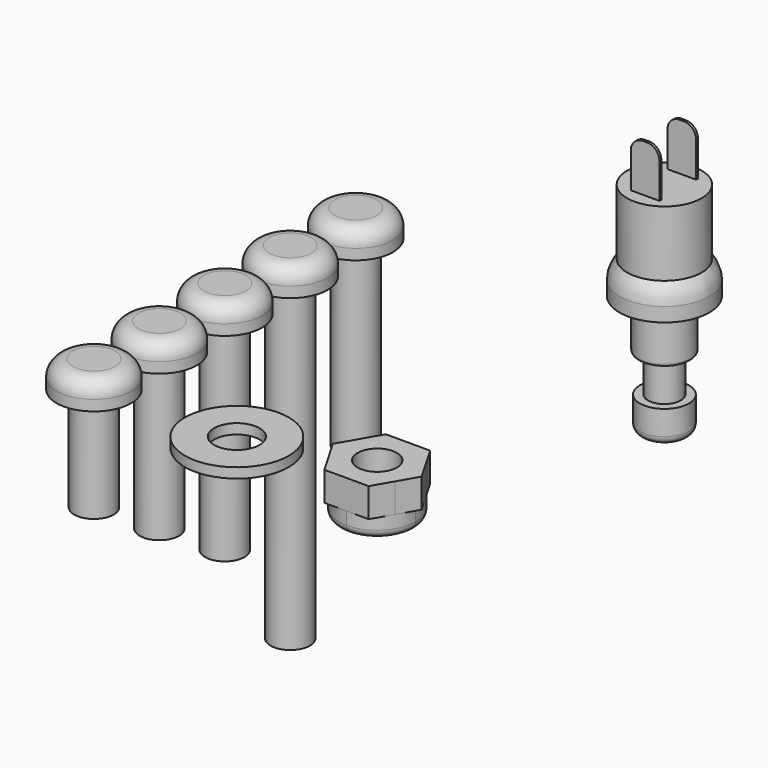
from build123d import *

# Parameters (mm, degrees)
F0_R      = 3
F1_DEPTH  = 4
F2_R      = 2
F3_DEPTH  = 4.6
F4_R      = 3.175
F5_DEPTH  = 6
F6_R      = 5.5
F7_DEPTH  = 4
F8_R      = 4.5612364212
F9_DEPTH  = 8
F11_R     = 1
F12_R     = 0.3
F13_W     = 3.5
F13_H     = 0.3
F14_DEPTH = 5.8
F15_R     = 1.5
F16_R     = 4.57
F16_R_2   = 2.413
F17_DEPTH = 3.3
F18_R     = 2
F19_DEPTH = 1
F21_DEPTH = 11.7
F23_DEPTH = 18.05
F25_DEPTH = 24.4
F27_DEPTH = 38
F28_R     = 6.35
F28_R_2   = 2.78
F29_DEPTH = 1.225
F30_R     = 2.413
F31_DEPTH = 3.56
F32_DEPTH = 2.54
F33_R     = 1
F34_DEPTH = 21.225


# Not quite as in the source:
# - a fillet or chamfer that OpenCascade refuses, or shapes differently, is made with other operations: its cross-section is extruded or revolved along the edge and cut away or added


with BuildPart() as f1:
    # F0 (on Top) → F1 (new body)
    with BuildSketch(Plane.XY):
        Circle(F0_R)
    extrude(amount=F1_DEPTH)

    # F2 (on face) → F3 (join)
    with BuildSketch(Plane.XY.offset(4)):
        Circle(F2_R)
    extrude(amount=F3_DEPTH)

    # F4 (on face) → F5 (join)
    with BuildSketch(Plane.XY.offset(8.6)):
        Circle(F4_R)
    extrude(amount=F5_DEPTH)

    # F6 (on face) → F7 (join)
    with BuildSketch(Plane.XY.offset(14.6)):
        Circle(F6_R)
    extrude(amount=F7_DEPTH)

    # F8 (on face) → F9 (join)
    with BuildSketch(Plane.XY.offset(18.6)):
        Circle(F8_R)
    extrude(amount=F9_DEPTH)

    # F10: fillet of radius 3.2064860271 on 1 edges, made by hand

    # F10_s1 → F10_t2 (revolve, cut)
    with BuildSketch(Plane.XZ):
        with BuildLine():
            ThreePointArc((5.5, 16.3330664898), (5.256027516, 17.5598778645), (4.5612364212, 18.6))
            Line((4.5612364212, 18.6), (5.5, 18.6))
            Line((5.5, 18.6), (5.5, 16.3330664898))
        make_face()
    revolve(axis=Axis((0, 0, 18.6), (0, 0, 1)), mode=Mode.SUBTRACT)

    # F11
    f11_edges = [f1.edges().sort_by_distance(p)[0] for p in [
        (-3, 0, 0),
    ]]
    fillet(f11_edges, radius=F11_R)

    # F12
    f12_edges = [f1.edges().sort_by_distance(p)[0] for p in [
        (-3.175, 0, 8.6),
    ]]
    fillet(f12_edges, radius=F12_R)

    # F13 (on face) → F14 (join)
    with BuildSketch(Plane.XY.offset(26.6)):
        with Locations((0, 2.8059364047)):
            Rectangle(F13_W, F13_H)
        with Locations((0, -2.8059364047)):
            Rectangle(F13_W, F13_H)
    extrude(amount=F14_DEPTH)

    # F15
    f15_edges = [f1.edges().sort_by_distance(p)[0] for p in [
        (1.75, 2.805936, 32.4),
        (1.75, -2.805936, 32.4),
        (-1.75, -2.805936, 32.4),
        (-1.75, 2.805936, 32.4),
    ]]
    fillet(f15_edges, radius=F15_R)


with BuildPart() as f17:
    # F16 (on Top) → F17 (new body)
    with BuildSketch(Plane.XY):
        with Locations((-47.9814447463, -27.2121559829)):
            Circle(F16_R)
        with Locations((-47.9814447463, -27.2121559829)):
            Circle(F16_R_2, mode=Mode.SUBTRACT)
        with Locations((-47.9814447463, -27.2121559829)):
            Circle(F16_R_2)
    extrude(amount=F17_DEPTH)

    # F18
    f18_edges = [f17.edges().sort_by_distance(p)[0] for p in [
        (-52.551445, -27.212156, 3.3),
    ]]
    fillet(f18_edges, radius=F18_R)

    # F16 (on Top) → F19 (join)
    with BuildSketch(Plane.XY):
        with Locations((-47.9814447463, -27.2121559829)):
            Circle(F16_R_2)
    extrude(amount=-F19_DEPTH)


with BuildPart() as f20_1:
    # F20: copy of F17
    add(f17.part.moved(Location((0, 10, 0))))


with BuildPart() as f17_1:
    add(f17.part)

    # F21 (add): a face of the model
    f21_faces = [f17_1.faces().sort_by_distance(p)[0] for p in [
        (-47.9814447463, -27.2121559829, -1),
    ]]
    extrude(f21_faces, amount=F21_DEPTH)


with BuildPart() as f22_1:
    # F22: copy of F20_1
    add(f20_1.part.moved(Location((0, 10, 0))))


with BuildPart() as f20_1_1:
    add(f20_1.part)

    # F23 (add): a face of the model
    f23_faces = [f20_1_1.faces().sort_by_distance(p)[0] for p in [
        (-47.9814447463, -17.2121559829, -1),
    ]]
    extrude(f23_faces, amount=F23_DEPTH)


with BuildPart() as f24_1:
    # F24: copy of F22_1
    add(f22_1.part.moved(Location((0, 10, 0))))


with BuildPart() as f22_1_1:
    add(f22_1.part)

    # F25 (add): a face of the model
    f25_faces = [f22_1_1.faces().sort_by_distance(p)[0] for p in [
        (-47.9814447463, -7.2121559829, -1),
    ]]
    extrude(f25_faces, amount=F25_DEPTH)


with BuildPart() as f26_1:
    # F26: copy of F24_1
    add(f24_1.part.moved(Location((0, 10, 0))))

    # F34 (add): a face of the model
    f34_faces = [f26_1.faces().sort_by_distance(p)[0] for p in [
        (-47.9814447463, 12.7878440171, -1),
    ]]
    extrude(f34_faces, amount=F34_DEPTH)


with BuildPart() as f24_1_1:
    add(f24_1.part)

    # F27 (add): a face of the model
    f27_faces = [f24_1_1.faces().sort_by_distance(p)[0] for p in [
        (-47.9814447463, 2.7878440171, -1),
    ]]
    extrude(f27_faces, amount=F27_DEPTH)


with BuildPart() as f29:
    # F28 (on Top) → F29 (new body)
    with BuildSketch(Plane.XY):
        with Locations((-29.7613665462, -28.1460825354)):
            Circle(F28_R)
        with Locations((-29.7613665462, -28.1460825354)):
            Circle(F28_R_2, mode=Mode.SUBTRACT)
    extrude(amount=F29_DEPTH)


with BuildPart() as f31:
    # F30 (on Top) → F31 (new body)
    with BuildSketch(Plane.XY):
        with BuildLine():
            Line((-13.4401228279, -22.3916537771), (-16.1530917428, -22.3916537771))
            Line((-16.1530917428, -22.3916537771), (-17.5095760985, -24.7411536008))
            ThreePointArc((-17.5095760985, -24.7411536008), (-15.7896227397, -23.0212003538), (-13.4401228279, -22.3916537771))
        make_face()
        with BuildLine():
            Line((-10.727153913, -22.3916537771), (-13.4401228279, -22.3916537771))
            ThreePointArc((-13.4401228279, -22.3916537771), (-11.0906228488, -23.0212003927), (-9.3706694796, -24.7411537354))
            Line((-9.3706694796, -24.7411537354), (-10.727153913, -22.3916537771))
        make_face()
        with BuildLine():
            ThreePointArc((-9.3706694796, -24.7411537354), (-11.0906228488, -23.0212003927), (-13.4401228279, -22.3916537771))
            ThreePointArc((-13.4401228279, -22.3916537771), (-15.7896227397, -23.0212003538), (-17.5095760985, -24.7411536008))
            ThreePointArc((-17.5095760985, -24.7411536008), (-18.1391228279, -27.0906535737), (-17.5095763019, -29.4401536012))
            ThreePointArc((-17.5095763019, -29.4401536012), (-15.7896229159, -31.1601070987), (-13.4401228279, -31.7896537771))
            ThreePointArc((-13.4401228279, -31.7896537771), (-11.0906228488, -31.1601071616), (-9.3706694796, -29.4401538189))
            ThreePointArc((-9.3706694796, -29.4401538189), (-8.9012373764, -28.3068444934), (-8.7411228279, -27.0906537771))
            ThreePointArc((-8.7411228279, -27.0906537771), (-8.9012373764, -25.8744630609), (-9.3706694796, -24.7411537354))
        make_face()
        with Locations((-13.4401228279, -27.0906537771)):
            Circle(F30_R, mode=Mode.SUBTRACT)
        with BuildLine():
            ThreePointArc((-17.5095763019, -29.4401536012), (-18.1391228279, -27.0906535737), (-17.5095760985, -24.7411536008))
            Line((-17.5095760985, -24.7411536008), (-18.8660606577, -27.0906537771))
            Line((-18.8660606577, -27.0906537771), (-17.5095763019, -29.4401536012))
        make_face()
        with BuildLine():
            Line((-8.014184998, -27.0906537771), (-9.3706694796, -24.7411537354))
            ThreePointArc((-9.3706694796, -24.7411537354), (-8.9012373764, -25.8744630609), (-8.7411228279, -27.0906537771))
            ThreePointArc((-8.7411228279, -27.0906537771), (-8.9012373764, -28.3068444934), (-9.3706694796, -29.4401538189))
            Line((-9.3706694796, -29.4401538189), (-8.014184998, -27.0906537771))
        make_face()
        with BuildLine():
            ThreePointArc((-13.4401228279, -31.7896537771), (-15.7896229159, -31.1601070987), (-17.5095763019, -29.4401536012))
            Line((-17.5095763019, -29.4401536012), (-16.1530917428, -31.7896537771))
            Line((-16.1530917428, -31.7896537771), (-13.4401228279, -31.7896537771))
        make_face()
        with BuildLine():
            ThreePointArc((-9.3706694796, -29.4401538189), (-11.0906228488, -31.1601071616), (-13.4401228279, -31.7896537771))
            Line((-13.4401228279, -31.7896537771), (-10.727153913, -31.7896537771))
            Line((-10.727153913, -31.7896537771), (-9.3706694796, -29.4401538189))
        make_face()
    extrude(amount=F31_DEPTH)

    # F30 (on Top) → F32 (join)
    with BuildSketch(Plane.XY):
        with BuildLine():
            ThreePointArc((-9.3706694796, -24.7411537354), (-11.0906228488, -23.0212003927), (-13.4401228279, -22.3916537771))
            ThreePointArc((-13.4401228279, -22.3916537771), (-15.7896227397, -23.0212003538), (-17.5095760985, -24.7411536008))
            ThreePointArc((-17.5095760985, -24.7411536008), (-18.1391228279, -27.0906535737), (-17.5095763019, -29.4401536012))
            ThreePointArc((-17.5095763019, -29.4401536012), (-15.7896229159, -31.1601070987), (-13.4401228279, -31.7896537771))
            ThreePointArc((-13.4401228279, -31.7896537771), (-11.0906228488, -31.1601071616), (-9.3706694796, -29.4401538189))
            ThreePointArc((-9.3706694796, -29.4401538189), (-8.9012373764, -28.3068444934), (-8.7411228279, -27.0906537771))
            ThreePointArc((-8.7411228279, -27.0906537771), (-8.9012373764, -25.8744630609), (-9.3706694796, -24.7411537354))
        make_face()
        with Locations((-13.4401228279, -27.0906537771)):
            Circle(F30_R, mode=Mode.SUBTRACT)
    extrude(amount=-F32_DEPTH)

    # F33
    f33_edges = [f31.edges().sort_by_distance(p)[0] for p in [
        (-9.370669, -24.741154, -2.54),
    ]]
    fillet(f33_edges, radius=F33_R)


solid = Compound([f1.part, f17_1.part, f20_1_1.part, f22_1_1.part, f26_1.part, f24_1_1.part, f29.part, f31.part])
